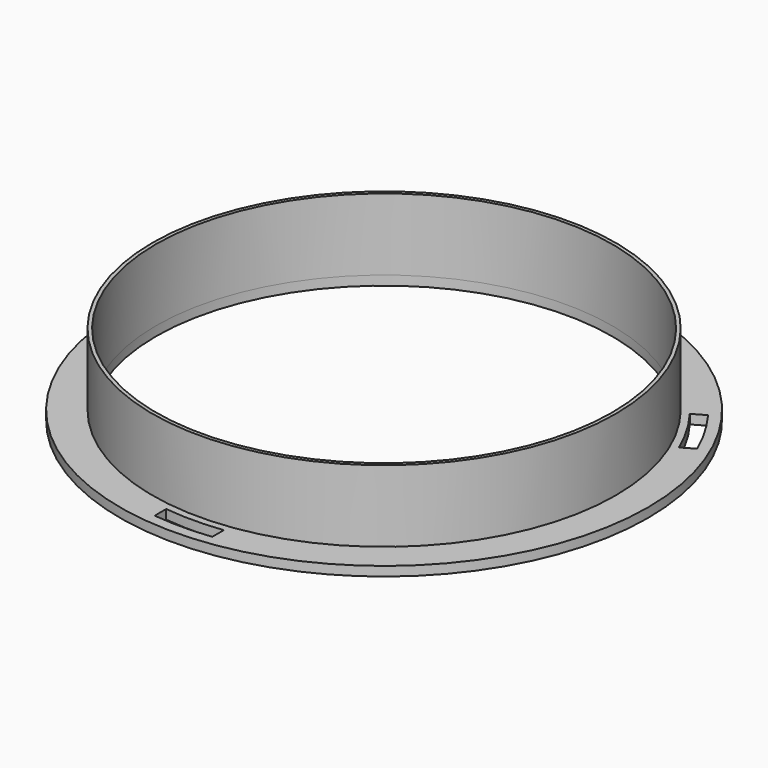
from build123d import *

# Parameters (mm, degrees)
F0_R     = 64.5
F0_R_2   = 63.5
F1_DEPTH = 20
F2_R     = 73.5
F2_R_2   = 64.5
F2_R_3   = 63.5
F3_DEPTH = 2.6


with BuildPart() as f1:
    # F0 (on Top) → F1 (new body)
    with BuildSketch(Plane.XY):
        Circle(F0_R)
        Circle(F0_R_2, mode=Mode.SUBTRACT)
    extrude(amount=F1_DEPTH)


with BuildPart() as f3:
    # F2 (on face) → F3 (new body)
    with BuildSketch(Plane(origin=(0, 0, 0), x_dir=(1, 0, 0), z_dir=(0, 0, -1))):
        Circle(F2_R)
        with BuildLine():
            Line((-53.272543663, -39.8030914839), (-56.759545298, -41.8163128165))
            ThreePointArc((-56.759545298, -41.8163128165), (-61.1380505803, -35.1053951871), (-64.7267495, -27.9409716932))
            Line((-64.7267495, -27.9409716932), (-61.2377470377, -25.9265951823))
            ThreePointArc((-61.2377470377, -25.9265951823), (-57.6740058995, -33.1052721407), (-53.272543663, -39.8030914839))
        make_face(mode=Mode.SUBTRACT)
        with BuildLine():
            Line((61.1067602057, -26.2338303944), (64.5937618407, -28.2470517271))
            ThreePointArc((64.5937618407, -28.2470517271), (60.971189332, -35.3944073469), (56.5609660427, -42.0845235248))
            Line((56.5609660427, -42.0845235248), (53.0719635804, -40.070147014))
            ThreePointArc((53.0719635804, -40.070147014), (57.5070096228, -33.3945181766), (61.1067602057, -26.2338303944))
        make_face(mode=Mode.SUBTRACT)
        Circle(F2_R_2, mode=Mode.SUBTRACT)
        with BuildLine():
            Line((-7.8342165427, 66.0369218783), (-7.8342165427, 70.0633645435))
            ThreePointArc((-7.8342165427, 70.0633645435), (0.1668612483, 70.4998025339), (8.1657834573, 70.025495218))
            Line((8.1657834573, 70.025495218), (8.1657834573, 65.9967421963))
            ThreePointArc((8.1657834573, 65.9967421963), (0.1669962767, 66.4997903173), (-7.8342165427, 66.0369218783))
        make_face(mode=Mode.SUBTRACT)
        Circle(F2_R_2)
        Circle(F2_R_3, mode=Mode.SUBTRACT)
    extrude(amount=F3_DEPTH)


solid = Compound([f1.part, f3.part])
